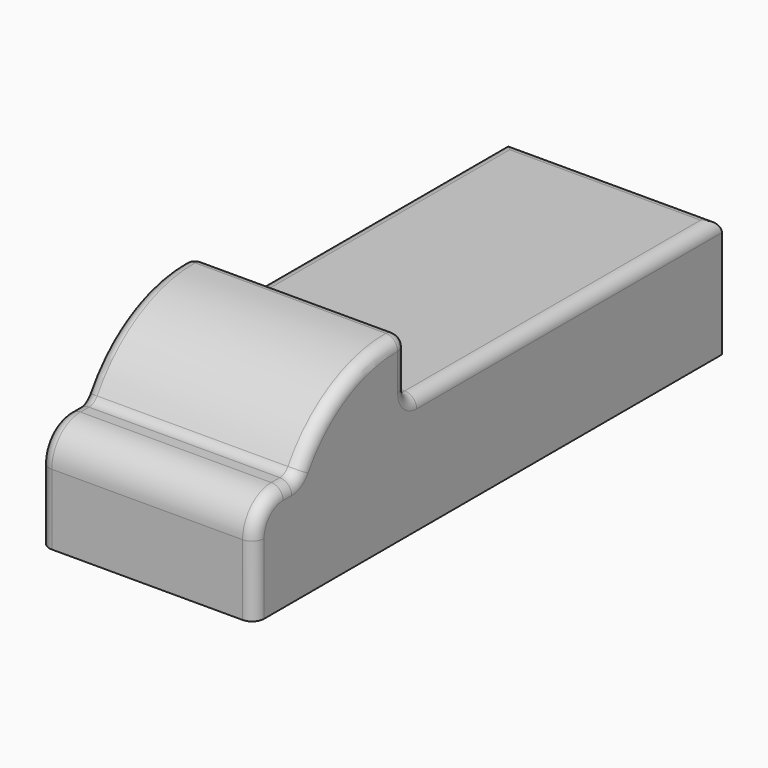
from build123d import *

# Parameters (mm, degrees)
F1_DEPTH = 90
F2_R     = 15
F3_R     = 5


with BuildPart() as f1:
    # F0 (on Right) → F1 (new body)
    with BuildSketch(Plane.YZ):
        with BuildLine():
            Line((0, 15), (0, 0))
            Line((0, 0), (245, 0))
            Line((245, 0), (245, 50))
            Line((245, 50), (80, 50))
            Line((80, 50), (80, 75))
            ThreePointArc((80, 75), (46.6250520012, 68.4603820444), (22.3636995256, 44.6267811209))
            Line((22.3636995256, 44.6267811209), (0, 44.6267811209))
            Line((0, 44.6267811209), (0, 15))
        make_face()
    extrude(amount=F1_DEPTH)

    # F2
    f2_edges = [f1.edges().sort_by_distance(p)[0] for p in [
        (45, 0, 44.626781),
    ]]
    fillet(f2_edges, radius=F2_R)

    # F3
    f3_edges = [f1.edges().sort_by_distance(p)[0] for p in [
        (90, 46.625052, 68.460382),
        (90, 162.5, 50),
        (90, 18.68185, 44.626781),
        (45, 22.3637, 44.626781),
        (0, 18.68185, 44.626781),
        (0, 80, 62.5),
        (0, 162.5, 50),
        (45, 245, 50),
        (90, 80, 62.5),
        (45, 80, 75),
        (45, 80, 50),
        (0, 4.393398, 40.233383),
        (0, 46.625052, 68.460382),
        (0, 0, 14.813391),
        (90, 4.393398, 40.233383),
        (90, 0, 14.813391),
    ]]
    fillet(f3_edges, radius=F3_R)


solid = f1.part
